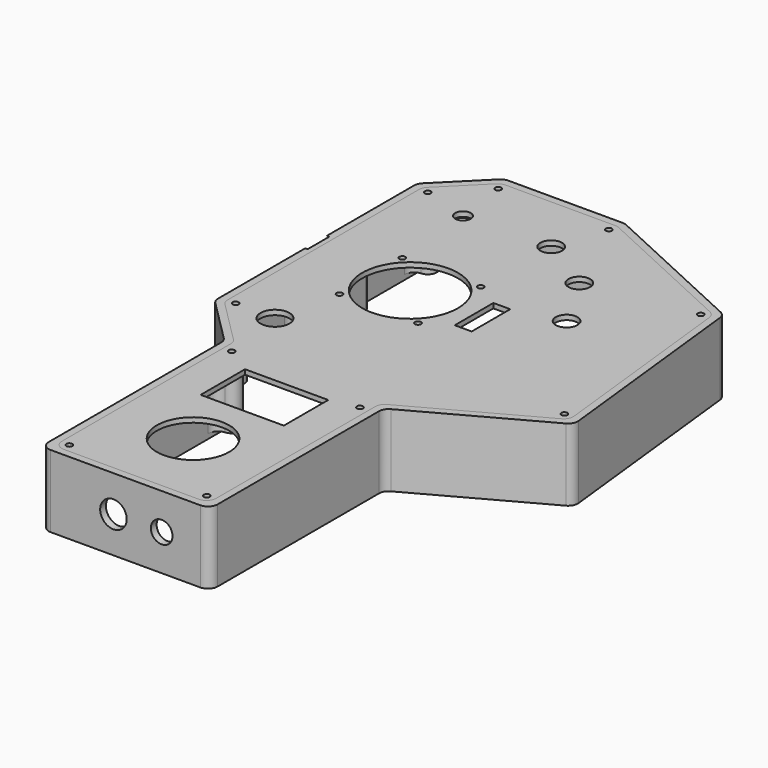
from build123d import *

# Parameters (mm, degrees)
F1_DEPTH    = 15
F2_R        = 4
F4_R        = 3.75
F4_R_2      = 1.25
F4_W        = 6
F4_H        = 32
F5_DEPTH    = 13
F6_T1_DEPTH = 26
F7_R        = 5.5
F7_R_2      = 4.5
F8_DEPTH    = 3
F10_DEPTH   = 1
F11_R       = 1
F11_R_2     = 4.5
F12_DEPTH   = 8.5
F13_R       = 1.5
F14_R       = 3.25
F15_DEPTH   = 3
F16_R       = 2
F18_DEPTH   = 2
F19_DEPTH   = 25
F20_R       = 19.85
F20_W       = 7
F20_H       = 20
F20_R_2     = 4.5
F20_R_3     = 3.25
F20_R_4     = 6
F20_W_2     = 34.5
F20_H_2     = 23
F20_R_5     = 15
F20_R_6     = 1.25
F21_DEPTH   = 25


# Not quite as in the source:
# - a fillet or chamfer that OpenCascade refuses, or shapes differently, is made with other operations: its cross-section is extruded or revolved along the edge and cut away or added


with BuildPart() as f1:
    # F0 (on Top) → F1 (new body, symmetric)
    with BuildSketch(Plane.XY):
        Polygon((-16.4496773855, 92.8151577375), (-66.4496773855, 92.8151577375), (-86.4496773855, 72.8151577375), (-86.4496773855, -32.1848422625), (-66.4496773855, -52.1848422625), (-66.4496773855, -147.1848422625), (3.5503226145, -147.1848422625), (3.5503226145, -57.1848422625), (58.5503226145, -27.1848422625), (48.5503226145, 62.8151577375), align=None)
        Polygon((45.7556689461, 60.8008853391), (55.3463454544, -25.5152032355), (0.5503226145, -55.4039429663), (0.5503226145, -144.1848422625), (-63.4496773855, -144.1848422625), (-63.4496773855, -50.9422015754), (-83.4496773855, -30.9422015754), (-83.4496773855, 71.5725170504), (-65.2070366983, 89.8151577375), (-17.1085879171, 89.8151577375), align=None, mode=Mode.SUBTRACT)
    extrude(amount=F1_DEPTH, both=True)

    # F2
    f2_edges = [f1.edges().sort_by_distance(p)[0] for p in [
        (3.550323, -147.184842, 0),
        (-66.449677, -147.184842, 0),
        (-66.449677, -52.184842, 0),
        (-86.449677, -32.184842, 0),
        (-86.449677, 72.815158, 0),
        (-66.449677, 92.815158, 0),
        (-16.449677, 92.815158, 0),
        (48.550323, 62.815158, 0),
        (58.550323, -27.184842, 0),
        (3.550323, -57.184842, 0),
        (-83.449677, 71.572517, 0),
        (-65.207037, 89.815158, 0),
        (-17.108588, 89.815158, 0),
        (45.755669, 60.800885, 0),
        (55.346345, -25.515203, 0),
        (0.550323, -55.403943, 0),
        (-63.449677, -50.942202, 0),
        (-83.449677, -30.942202, 0),
        (-63.449677, -144.184842, 0),
        (0.550323, -144.184842, 0),
    ]]
    fillet(f2_edges, radius=F2_R)

    # F4 (on Top) → F5 (join, symmetric)
    with BuildSketch(Plane.XY):
        with Locations((-59.9496773855, -140.6848422625)):
            Circle(F4_R)
        with Locations((-59.9496773855, -140.6848422625)):
            Circle(F4_R_2, mode=Mode.SUBTRACT)
        with Locations((-2.9496773855, -140.6848422625)):
            Circle(F4_R)
        with Locations((-2.9496773855, -140.6848422625)):
            Circle(F4_R_2, mode=Mode.SUBTRACT)
        with Locations((-2.9496773855, -61.2943926144)):
            Circle(F4_R)
        with Locations((-2.9496773855, -61.2943926144)):
            Circle(F4_R_2, mode=Mode.SUBTRACT)
        with Locations((-59.9496773855, -56.563521919)):
            Circle(F4_R)
        with Locations((-59.9496773855, -56.563521919)):
            Circle(F4_R_2, mode=Mode.SUBTRACT)
        with Locations((-79.9496773855, -29.4924541071)):
            Circle(F4_R)
        with Locations((-79.9496773855, -29.4924541071)):
            Circle(F4_R_2, mode=Mode.SUBTRACT)
        with Locations((51.6083721009, -23.5672910373)):
            Circle(F4_R)
        with Locations((51.6083721009, -23.5672910373)):
            Circle(F4_R_2, mode=Mode.SUBTRACT)
        with Locations((42.4952396662, 58.4509008743)):
            Circle(F4_R)
        with Locations((42.4952396662, 58.4509008743)):
            Circle(F4_R_2, mode=Mode.SUBTRACT)
        with Locations((-17.8773168707, 86.3151577375)):
            Circle(F4_R)
        with Locations((-17.8773168707, 86.3151577375)):
            Circle(F4_R_2, mode=Mode.SUBTRACT)
        with Locations((-63.75728923, 86.3151577375)):
            Circle(F4_R)
        with Locations((-63.75728923, 86.3151577375)):
            Circle(F4_R_2, mode=Mode.SUBTRACT)
        with Locations((-79.9496773855, 70.1227695821)):
            Circle(F4_R)
        with Locations((-79.9496773855, 70.1227695821)):
            Circle(F4_R_2, mode=Mode.SUBTRACT)
        with Locations((-80.4496773855, 20.3151577375)):
            Rectangle(F4_W, F4_H)
    extrude(amount=F5_DEPTH, both=True)

    # F6: fillet of radius 4 on 18 edges, made by hand

    # F6_s2 → F6_t1 (join)
    with BuildSketch(Plane.XY.offset(-13)):
        with BuildLine():
            ThreePointArc((-63.9224059749, -50.712695203), (-62.3516704174, -52.3151692655), (-60.1652211816, -52.8197215942))
            Line((-60.1652211816, -52.8197215942), (-60.1422298434, -53.2190602955))
            ThreePointArc((-60.1422298434, -53.2190602955), (-61.9247985819, -53.8577140434), (-63.0763440521, -55.360835112))
            Line((-63.0763440521, -55.360835112), (-63.8496773855, -55.2172307172))
            ThreePointArc((-63.8496773855, -55.2172307172), (-63.8496773855, -52.5990558249), (-64.2751331159, -50.9013312652))
            Line((-64.2751331159, -50.9013312652), (-63.9224059749, -50.712695203))
        make_face()
        with BuildLine():
            ThreePointArc((-63.4496773855, -64.2973760681), (-62.3679181281, -61.5617096104), (-59.7077419016, -60.3057094105))
            ThreePointArc((-59.7077419016, -60.3057094105), (-61.9717619177, -59.7216343527), (-63.4496773855, -57.9098131207))
            Line((-63.4496773855, -57.9098131207), (-63.4496773855, -64.2973760681))
        make_face()
        with BuildLine():
            ThreePointArc((-83.4496773855, 62.3889154329), (-82.3679181281, 65.1245818906), (-79.7077419016, 66.3805820905))
            ThreePointArc((-79.7077419016, 66.3805820905), (-81.9717619177, 66.9646571483), (-83.4496773855, 68.7764783803))
            Line((-83.4496773855, 68.7764783803), (-83.4496773855, 62.3889154329))
        make_face()
        with BuildLine():
            ThreePointArc((-25.6111710198, 89.8151577375), (-22.8755045621, 88.7333984802), (-21.6195043622, 86.0732222536))
            ThreePointArc((-21.6195043622, 86.0732222536), (-21.0354293045, 88.3372422697), (-19.2236080725, 89.8151577375))
            Line((-19.2236080725, 89.8151577375), (-25.6111710198, 89.8151577375))
        make_face()
        with BuildLine():
            ThreePointArc((-60.0151017385, 86.0732222536), (-58.7591015386, 88.7333984802), (-56.0234350809, 89.8151577375))
            Line((-56.0234350809, 89.8151577375), (-62.4109980282, 89.8151577375))
            ThreePointArc((-62.4109980282, 89.8151577375), (-60.5991767963, 88.3372422697), (-60.0151017385, 86.0732222536))
        make_face()
        with BuildLine():
            ThreePointArc((42.6680393995, 54.7048842897), (45.4506473013, 53.7503334406), (46.8278940537, 51.1508593704))
            Line((46.8278940537, 51.1508593704), (46.1225057296, 57.499354288))
            ThreePointArc((46.1225057296, 57.499354288), (44.8537117686, 55.5354061748), (42.6680393995, 54.7048842897))
        make_face()
        with BuildLine():
            ThreePointArc((46.4948382392, -30.3432980801), (48.3784649861, -28.0836467051), (48.2072709471, -25.1468514008))
            ThreePointArc((48.2072709471, -25.1468514008), (49.8041586632, -26.854738964), (52.1024514723, -27.2845999529))
            Line((52.1024514723, -27.2845999529), (46.4948382392, -30.3432980801))
        make_face()
        with BuildLine():
            ThreePointArc((50.9546608831, -19.874709062), (53.4598647472, -18.3326235723), (54.2329038561, -15.4942288508))
            Line((54.2329038561, -15.4942288508), (54.9382921803, -21.8427237684))
            ThreePointArc((54.9382921803, -21.8427237684), (53.269333852, -20.2051925763), (50.9546608831, -19.874709062))
        make_face()
        with BuildLine():
            ThreePointArc((-76.9558904061, -37.4359885548), (-78.1253794029, -34.736660945), (-77.1324770125, -31.9675060376))
            ThreePointArc((-77.1324770125, -31.9675060376), (-79.1463843527, -33.1554065097), (-81.4725794814, -32.9192994795))
            Line((-81.4725794814, -32.9192994795), (-76.9558904061, -37.4359885548))
        make_face()
        with BuildLine():
            ThreePointArc((-79.7077419016, -25.7502666156), (-82.3679181281, -24.4942664157), (-83.4496773855, -21.758599958))
            Line((-83.4496773855, -21.758599958), (-83.4496773855, -28.1461629053))
            ThreePointArc((-83.4496773855, -28.1461629053), (-81.9717619177, -26.3343416733), (-79.7077419016, -25.7502666156))
        make_face()
        with BuildLine():
            ThreePointArc((-63.4496773855, -132.9509881134), (-62.3679181281, -135.6866545711), (-59.7077419016, -136.942654771))
            ThreePointArc((-59.7077419016, -136.942654771), (-61.9717619177, -137.5267298287), (-63.4496773855, -139.3385510607))
            Line((-63.4496773855, -139.3385510607), (-63.4496773855, -132.9509881134))
        make_face()
        with BuildLine():
            ThreePointArc((-56.2074898939, -140.4429067786), (-54.951489694, -143.1030830052), (-52.2158232363, -144.1848422625))
            Line((-52.2158232363, -144.1848422625), (-58.6033861837, -144.1848422625))
            ThreePointArc((-58.6033861837, -144.1848422625), (-56.7915649517, -142.7069267948), (-56.2074898939, -140.4429067786))
        make_face()
        with BuildLine():
            ThreePointArc((-10.6835315346, -144.1848422625), (-7.9478650769, -143.1030830052), (-6.691864877, -140.4429067786))
            ThreePointArc((-6.691864877, -140.4429067786), (-6.1077898192, -142.7069267948), (-4.2959685872, -144.1848422625))
            Line((-4.2959685872, -144.1848422625), (-10.6835315346, -144.1848422625))
        make_face()
        with BuildLine():
            ThreePointArc((-3.1916128693, -136.942654771), (-0.5314366428, -135.6866545711), (0.5503226145, -132.9509881134))
            Line((0.5503226145, -132.9509881134), (0.5503226145, -139.3385510607))
            ThreePointArc((0.5503226145, -139.3385510607), (-0.9275928532, -137.5267298287), (-3.1916128693, -136.942654771))
        make_face()
        with BuildLine():
            ThreePointArc((0.5503226145, -69.0282467635), (-0.5314366428, -66.2925803058), (-3.1916128693, -65.0365801059))
            ThreePointArc((-3.1916128693, -65.0365801059), (-0.9275928532, -64.4525050482), (0.5503226145, -62.6406838162))
            Line((0.5503226145, -62.6406838162), (0.5503226145, -69.0282467635))
        make_face()
        with BuildLine():
            ThreePointArc((1.1468493037, -55.6769593793), (-0.4663480378, -57.1524410146), (-2.6143289766, -57.5594171868))
            Line((-2.6143289766, -57.5594171868), (-2.6500994735, -57.9578145658))
            ThreePointArc((-2.6500994735, -57.9578145658), (-0.9314700284, -58.6205678138), (0.1769892812, -60.0917058075))
            Line((0.1769892812, -60.0917058075), (0.9503226145, -59.9481014126))
            ThreePointArc((0.9503226145, -59.9481014126), (0.9503226145, -57.7784753613), (1.4871966348, -55.8871109775))
            Line((1.4871966348, -55.8871109775), (1.1468493037, -55.6769593793))
        make_face()
        with BuildLine():
            ThreePointArc((-83.4496773855, 0.3151577375), (-82.2781045102, 3.1435848622), (-79.4496773855, 4.3151577375))
            Line((-79.4496773855, 4.3151577375), (-83.4496773855, 4.3151577375))
            Line((-83.4496773855, 4.3151577375), (-83.4496773855, 0.3151577375))
        make_face()
        with BuildLine():
            ThreePointArc((-83.4496773855, 40.3151577375), (-82.2781045102, 37.4867306127), (-79.4496773855, 36.3151577375))
            Line((-79.4496773855, 36.3151577375), (-83.4496773855, 36.3151577375))
            Line((-83.4496773855, 36.3151577375), (-83.4496773855, 40.3151577375))
        make_face()
    extrude(amount=F6_T1_DEPTH)

    # F7 (on face) → F8 (cut)
    with BuildSketch(Plane.XZ.offset(147.1848422625)):
        with Locations((-36.4496773855, 0)):
            Circle(F7_R)
        with Locations((-16.4496773855, 0)):
            Circle(F7_R_2)
    extrude(amount=-F8_DEPTH, mode=Mode.SUBTRACT)

    # F9 (on face) → F10 (cut)
    with BuildSketch(Plane(origin=(-86.4496773855, 0, 0), x_dir=(0, -1, 0), z_dir=(-1, 0, 0))):
        with BuildLine():
            ThreePointArc((-14.7473933747, -15), (-7.1796290118, -9.1355287257), (-4.3151577375, 0))
            ThreePointArc((-4.3151577375, 0), (-7.1796290118, 9.1355287257), (-14.7473933747, 15))
            Line((-14.7473933747, 15), (-25.8829221003, 15))
            ThreePointArc((-25.8829221003, 15), (-36.3151577375, 0), (-25.8829221003, -15))
            Line((-25.8829221003, -15), (-14.7473933747, -15))
        make_face()
    extrude(amount=-F10_DEPTH, mode=Mode.SUBTRACT)

    # F11 (on face) → F12 (cut)
    with BuildSketch(Plane(origin=(-85.4496773855, 0, 0), x_dir=(0, -1, 0), z_dir=(-1, 0, 0))):
        with Locations((-26.5651577375, 6.25)):
            Circle(F11_R)
        with Locations((-14.0651577375, 6.25)):
            Circle(F11_R)
        with Locations((-20.3151577375, 0)):
            Circle(F11_R_2)
        with Locations((-14.0651577375, -6.25)):
            Circle(F11_R)
        with Locations((-26.5651577375, -6.25)):
            Circle(F11_R)
    extrude(amount=-F12_DEPTH, mode=Mode.SUBTRACT)

    # F13
    f13_edges = [f1.edges().sort_by_distance(p)[0] for p in [
        (-77.449677, 4.315158, 0),
        (-77.449677, 36.315158, 0),
    ]]
    fillet(f13_edges, radius=F13_R)

    # F14 (on face) → F15 (cut)
    with BuildSketch(Plane(origin=(-79.6324175615, 79.6324175615, 0), x_dir=(-0.7071067812, -0.7071067812, 0), z_dir=(-0.7071067812, 0.7071067812, 0))):
        with Locations((-4.5010743224, 0)):
            Circle(F14_R)
    extrude(amount=-F15_DEPTH, mode=Mode.SUBTRACT)

    # F16
    f16_edges = [f1.edges().sort_by_distance(p)[0] for p in [
        (-67.184135, 87.83806, 0),
        (-81.472579, 73.549615, 0),
        (42.739566, 62.192933, 0),
        (-15.188236, 88.928841, 0),
    ]]
    fillet(f16_edges, radius=F16_R)


with BuildPart() as f18:
    # F17 (on face) → F18 (new body)
    with BuildSketch(Plane.XY.offset(13)):
        with BuildLine():
            Line((-17.9871352926, 89.8151577375), (-63.5501824488, 89.8151577375))
            ThreePointArc((-63.5501824488, 89.8151577375), (-65.0809161783, 89.5106758675), (-66.3786095736, 88.6435848622))
            Line((-66.3786095736, 88.6435848622), (-82.2781045102, 72.7440899256))
            ThreePointArc((-82.2781045102, 72.7440899256), (-83.1451955155, 71.4463965303), (-83.4496773855, 69.9156628009))
            Line((-83.4496773855, 69.9156628009), (-83.4496773855, -29.2853473259))
            ThreePointArc((-83.4496773855, -29.2853473259), (-83.1451955155, -30.8160810554), (-82.2781045102, -32.1137744506))
            Line((-82.2781045102, -32.1137744506), (-64.6212502607, -49.7706287001))
            ThreePointArc((-64.6212502607, -49.7706287001), (-63.7541592554, -51.0683220954), (-63.4496773855, -52.5990558249))
            Line((-63.4496773855, -52.5990558249), (-63.4496773855, -140.1848422625))
            ThreePointArc((-63.4496773855, -140.1848422625), (-62.2781045102, -143.0132693873), (-59.4496773855, -144.1848422625))
            Line((-59.4496773855, -144.1848422625), (-3.4496773855, -144.1848422625))
            ThreePointArc((-3.4496773855, -144.1848422625), (-0.6212502607, -143.0132693873), (0.5503226145, -140.1848422625))
            Line((0.5503226145, -140.1848422625), (0.5503226145, -57.7784753613))
            ThreePointArc((0.5503226145, -57.7784753613), (1.1107271375, -55.7366176398), (2.6349140918, -54.2668930696))
            Line((2.6349140918, -54.2668930696), (52.9897844302, -26.8006001577))
            ThreePointArc((52.9897844302, -26.8006001577), (54.6216235074, -25.1375401043), (55.0499108462, -22.8472917618))
            Line((55.0499108462, -22.8472917618), (46.0049989935, 58.5569149122))
            ThreePointArc((46.0049989935, 58.5569149122), (45.2744327955, 60.4540299465), (43.7056967647, 61.7470263459))
            Line((43.7056967647, 61.7470263459), (-16.3109025828, 89.4469952755))
            ThreePointArc((-16.3109025828, 89.4469952755), (-17.1290415192, 89.7220330972), (-17.9871352926, 89.8151577375))
        make_face()
    extrude(amount=F18_DEPTH)

    # F4 (on Top) → F19 (cut)
    with BuildSketch(Plane.XY):
        with Locations((-79.9496773855, 70.1227695821)):
            Circle(F4_R_2)
        with Locations((-79.9496773855, -29.4924541071)):
            Circle(F4_R_2)
        with Locations((-59.9496773855, -56.563521919)):
            Circle(F4_R_2)
        with Locations((-2.9496773855, -61.2943926144)):
            Circle(F4_R_2)
        with Locations((51.6083721009, -23.5672910373)):
            Circle(F4_R_2)
        with Locations((-59.9496773855, -140.6848422625)):
            Circle(F4_R_2)
        with Locations((-2.9496773855, -140.6848422625)):
            Circle(F4_R_2)
        with Locations((-17.8773168707, 86.3151577375)):
            Circle(F4_R_2)
        with Locations((-63.75728923, 86.3151577375)):
            Circle(F4_R_2)
        with Locations((42.4952396662, 58.4509008743)):
            Circle(F4_R_2)
    extrude(amount=F19_DEPTH, mode=Mode.SUBTRACT)

    # F20 (on face) → F21 (cut)
    with BuildSketch(Plane.XY.offset(15)):
        with Locations((-41.4496773855, 12.8151577375)):
            Circle(F20_R)
        with Locations((-11.4496773855, 12.8151577375)):
            Rectangle(F20_W, F20_H)
        with Locations((11.4994139859, 27.694462928)):
            Circle(F20_R_2)
        with Locations((-1.9616638659, 51.0995773919)):
            Circle(F20_R_2)
        with Locations((-24.9390266286, 65.2784631193)):
            Circle(F20_R_2)
        with Locations((-60.7381012467, 64.3220184936)):
            Circle(F20_R_3)
        with Locations((-63.4496773855, -29.7289981398)):
            Circle(F20_R_4)
        with Locations((-31.4496773855, -75.1848422625)):
            Rectangle(F20_W_2, F20_H_2)
        with Locations((-31.4496773855, -112.1848422625)):
            Circle(F20_R_5)
        with Locations((-57.6996773855, 29.0651577375)):
            Circle(F20_R_6)
        with Locations((-25.1996773855, 29.0651577375)):
            Circle(F20_R_6)
        with Locations((-57.6996773855, -3.4348422625)):
            Circle(F20_R_6)
        with Locations((-25.1996773855, -3.4348422625)):
            Circle(F20_R_6)
    extrude(amount=-F21_DEPTH, mode=Mode.SUBTRACT)


solid = Compound([f1.part, f18.part])
